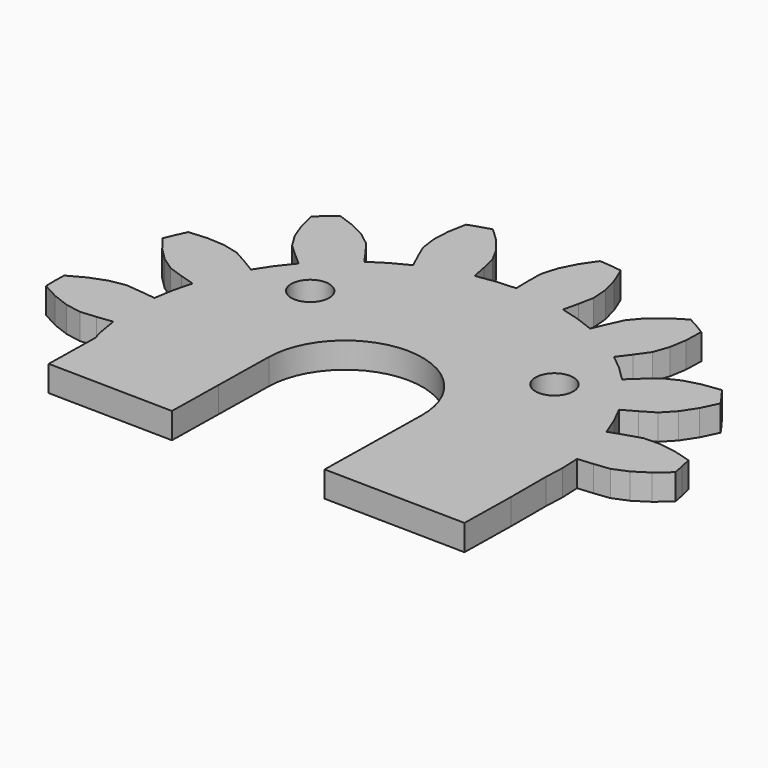
from build123d import *

# Parameters (mm, degrees)
F1_DEPTH  = 1.5
F2_R      = 1.1
F3_DEPTH  = 1.5
F4_W      = 4.2642379355
F4_H      = 1.5
F4_W_2    = 3
F4_W_3    = 5.2441455437
F3_FACE_W = 8.0745559603
F3_FACE_H = 1.5
F5_DEPTH  = 3.3


with BuildPart() as f1:
    # F0 (on Top) → F1 (new body)
    with BuildSketch(Plane.XY):
        Polygon((12.573339, -1.121183), (12.623723, 0), (12.573339, 1.121183), (13.469712, 1.201909), (14.363964, 1.305965), (15.232179, 1.665703), (16.071924, 2.205645), (16.876276, 2.889975), (16.752232, 3.534499), (16.603401, 4.173754), (15.590247, 4.47176), (14.603487, 4.623467), (13.664014, 4.59897), (12.804751, 4.330305), (11.95304, 4.039463), (11.543041, 5.084208), (11.040987, 6.087967), (11.82703, 6.526301), (12.601647, 6.985086), (13.248481, 7.666858), (13.796013, 8.501675), (14.252483, 9.454001), (13.877012, 9.992349), (13.481039, 10.515803), (12.434267, 10.375958), (11.471112, 10.113197), (10.622825, 9.7087), (9.947125, 9.113769), (9.287344, 8.50165), (8.487856, 9.28931), (7.620941, 10.002086), (8.16074, 10.722236), (8.681783, 11.456422), (8.995394, 12.342344), (9.156039, 13.327688), (9.185699, 14.383344), (8.623723, 14.722432), (8.049076, 15.039574), (7.149682, 14.486059), (6.376671, 13.854265), (5.766246, 13.139708), (5.390943, 12.321379), (5.037175, 11.493824), (3.986435, 11.888206), (2.904557, 12.186753), (3.104777, 13.0642), (3.282153, 13.946839), (3.208314, 14.883726), (2.954295, 15.849223), (2.552017, 16.825676), (1.900707, 16.906872), (1.246748, 16.962866), (0.650245, 16.091388), (0.201038, 15.199803), (-0.065977, 14.298742), (-0.075988, 13.398512), (-0.062575, 12.498612), (-1.182883, 12.431524), (-2.292658, 12.264221), (-2.466637, 13.147244), (-2.663598, 14.025721), (-3.112119, 14.851577), (-3.736881, 15.630283), (-4.501539, 16.358696), (-5.129566, 16.167961), (-5.749762, 15.953124), (-5.940233, 14.91437), (-5.987963, 13.917158), (-5.865399, 12.985393), (-5.508388, 12.15892), (-5.130112, 11.342276), (-6.126277, 10.825318), (-7.072058, 10.221092), (-7.590155, 10.957011), (-8.127396, 11.679428), (-8.873046, 12.251455), (-9.760523, 12.708725), (-10.755346, 13.063149), (-11.251497, 12.633462), (-11.730693, 12.184943), (-11.482197, 11.158522), (-11.120198, 10.22811), (-10.629247, 9.426751), (-9.966945, 8.81694), (-9.289213, 8.224757), (-9.988989, 7.347316), (-10.607243, 6.410645), (-11.379873, 6.872211), (-12.164501, 7.313656), (-13.07835, 7.532945), (-14.075089, 7.589713), (-15.128062, 7.508865), (-15.40655, 6.914523), (-15.661887, 6.309874), (-15.017392, 5.473264), (-14.308257, 4.770528), (-13.533809, 4.238139), (-12.680733, 3.950431), (-11.820732, 3.685104), (-12.103122, 2.598896), (-12.286947, 1.491738), (-13.180515, 1.599143), (-14.07686, 1.683286), (-15.000896, 1.511921), (-15.934551, 1.158371), (-16.863606, 0.656229), (-16.876277, 0), (-16.863606, -0.656229), (-15.934551, -1.158371), (-15.000896, -1.511921), (-14.07686, -1.683286), (-13.180515, -1.599143), (-12.286947, -1.491738), (-12.103122, -2.598896), (-11.820732, -3.685104), (-12.680733, -3.950431), (-13.533809, -4.238139), (-14.308257, -4.770528), (-15.017392, -5.473264), (-15.661887, -6.309874), (-15.40655, -6.914523), (-15.128062, -7.508865), (-14.075089, -7.589713), (-13.07835, -7.532945), (-12.164501, -7.313656), (-11.379873, -6.872211), (-10.607243, -6.410645), (-9.988989, -7.347316), (-9.289213, -8.224757), (-9.966945, -8.81694), (-10.629247, -9.426751), (-11.120198, -10.22811), (-11.482197, -11.158522), (-11.730693, -12.184943), (-11.251497, -12.633462), (-10.755346, -13.063149), (-9.760523, -12.708725), (-8.873046, -12.251455), (-8.127396, -11.679428), (-7.590155, -10.957011), (-7.072058, -10.221092), (-6.126277, -10.825318), (-5.130112, -11.342276), (-5.508388, -12.15892), (-5.865399, -12.985393), (-5.987963, -13.917158), (-5.940233, -14.91437), (-5.749762, -15.953124), (-5.129566, -16.167961), (-4.501539, -16.358696), (-3.736881, -15.630283), (-3.112119, -14.851577), (-2.663598, -14.025721), (-2.466637, -13.147244), (-2.292658, -12.264221), (-1.182883, -12.431524), (-0.062575, -12.498612), (-0.075988, -13.398512), (-0.065977, -14.298742), (0.201038, -15.199803), (0.650245, -16.091388), (1.246748, -16.962866), (1.900707, -16.906872), (2.552017, -16.825676), (2.954295, -15.849223), (3.208314, -14.883726), (3.282153, -13.946839), (3.104777, -13.0642), (2.904557, -12.186753), (3.986435, -11.888206), (5.037175, -11.493824), (5.390943, -12.321379), (5.766246, -13.139708), (6.376671, -13.854265), (7.149682, -14.486059), (8.049076, -15.039574), (8.623723, -14.722432), (9.185699, -14.383344), (9.156039, -13.327688), (8.995394, -12.342344), (8.681783, -11.456422), (8.16074, -10.722236), (7.620941, -10.002086), (8.487856, -9.28931), (9.287344, -8.50165), (9.947125, -9.113769), (10.622825, -9.7087), (11.471112, -10.113197), (12.434267, -10.375958), (13.481039, -10.515803), (13.877012, -9.992349), (14.252483, -9.454001), (13.796013, -8.501675), (13.248481, -7.666858), (12.601647, -6.985086), (11.82703, -6.526301), (11.040987, -6.087967), (11.543041, -5.084208), (11.95304, -4.039463), (12.804751, -4.330305), (13.664014, -4.59897), (14.603487, -4.623467), (15.590247, -4.47176), (16.603401, -4.173754), (16.752232, -3.534499), (16.876276, -2.889975), (16.071924, -2.205645), (15.232179, -1.665703), (14.363964, -1.305965), (13.469712, -1.201909), align=None)
    extrude(amount=F1_DEPTH)

    # F2 (on face) → F3 (cut, through all)
    with BuildSketch(Plane.XY.offset(1.5)):
        with Locations((-7.1978296976, 6.45)):
            Circle(F2_R)
        with Locations((7.2, 6.2)):
            Circle(F2_R)
        with BuildLine():
            Line((13.469712, -1.201909), (12.573339, -1.121183))
            Line((12.573339, -1.121183), (12.573339, -3.685104))
            Line((12.573339, -3.685104), (4.5, -3.5449207368))
            Line((4.5, -3.5449207368), (4.330384853, -3.5449207368))
            Line((4.330384853, -3.5449207368), (4.3927680428, 0.0478094358))
            ThreePointArc((4.3927680428, 0.0478094358), (-0.0284287377, 4.6252562163), (-4.6058755182, 0.2040594358))
            Line((-4.6058755182, 0.2040594358), (-4.6682075846, -3.3857264732))
            Line((-4.6682075846, -3.3857264732), (-11.9313506872, -3.2596112313))
            Line((-11.9313506872, -3.2596112313), (-11.820732, -3.685104))
            Line((-11.820732, -3.685104), (-12.680733, -3.950431))
            Line((-12.680733, -3.950431), (-13.533809, -4.238139))
            Line((-13.533809, -4.238139), (-14.308257, -4.770528))
            Line((-14.308257, -4.770528), (-15.017392, -5.473264))
            Line((-15.017392, -5.473264), (-15.661887, -6.309874))
            Line((-15.661887, -6.309874), (-15.40655, -6.914523))
            Line((-15.40655, -6.914523), (-15.128062, -7.508865))
            Line((-15.128062, -7.508865), (-14.075089, -7.589713))
            Line((-14.075089, -7.589713), (-13.07835, -7.532945))
            Line((-13.07835, -7.532945), (-12.164501, -7.313656))
            Line((-12.164501, -7.313656), (-11.379873, -6.872211))
            Line((-11.379873, -6.872211), (-10.607243, -6.410645))
            Line((-10.607243, -6.410645), (-9.988989, -7.347316))
            Line((-9.988989, -7.347316), (-9.289213, -8.224757))
            Line((-9.289213, -8.224757), (-9.966945, -8.81694))
            Line((-9.966945, -8.81694), (-10.629247, -9.426751))
            Line((-10.629247, -9.426751), (-11.120198, -10.22811))
            Line((-11.120198, -10.22811), (-11.482197, -11.158522))
            Line((-11.482197, -11.158522), (-11.730693, -12.184943))
            Line((-11.730693, -12.184943), (-11.251497, -12.633462))
            Line((-11.251497, -12.633462), (-10.755346, -13.063149))
            Line((-10.755346, -13.063149), (-9.760523, -12.708725))
            Line((-9.760523, -12.708725), (-8.873046, -12.251455))
            Line((-8.873046, -12.251455), (-8.127396, -11.679428))
            Line((-8.127396, -11.679428), (-7.590155, -10.957011))
            Line((-7.590155, -10.957011), (-7.072058, -10.221092))
            Line((-7.072058, -10.221092), (-6.126277, -10.825318))
            Line((-6.126277, -10.825318), (-5.130112, -11.342276))
            Line((-5.130112, -11.342276), (-5.508388, -12.15892))
            Line((-5.508388, -12.15892), (-5.865399, -12.985393))
            Line((-5.865399, -12.985393), (-5.987963, -13.917158))
            Line((-5.987963, -13.917158), (-5.940233, -14.91437))
            Line((-5.940233, -14.91437), (-5.749762, -15.953124))
            Line((-5.749762, -15.953124), (-5.129566, -16.167961))
            Line((-5.129566, -16.167961), (-4.501539, -16.358696))
            Line((-4.501539, -16.358696), (-3.736881, -15.630283))
            Line((-3.736881, -15.630283), (-3.112119, -14.851577))
            Line((-3.112119, -14.851577), (-2.663598, -14.025721))
            Line((-2.663598, -14.025721), (-2.466637, -13.147244))
            Line((-2.466637, -13.147244), (-2.292658, -12.264221))
            Line((-2.292658, -12.264221), (-1.182883, -12.431524))
            Line((-1.182883, -12.431524), (-0.062575, -12.498612))
            Line((-0.062575, -12.498612), (-0.075988, -13.398512))
            Line((-0.075988, -13.398512), (-0.065977, -14.298742))
            Line((-0.065977, -14.298742), (0.201038, -15.199803))
            Line((0.201038, -15.199803), (0.650245, -16.091388))
            Line((0.650245, -16.091388), (1.246748, -16.962866))
            Line((1.246748, -16.962866), (1.900707, -16.906872))
            Line((1.900707, -16.906872), (2.552017, -16.825676))
            Line((2.552017, -16.825676), (2.954295, -15.849223))
            Line((2.954295, -15.849223), (3.208314, -14.883726))
            Line((3.208314, -14.883726), (3.282153, -13.946839))
            Line((3.282153, -13.946839), (3.104777, -13.0642))
            Line((3.104777, -13.0642), (2.904557, -12.186753))
            Line((2.904557, -12.186753), (3.986435, -11.888206))
            Line((3.986435, -11.888206), (5.037175, -11.493824))
            Line((5.037175, -11.493824), (5.390943, -12.321379))
            Line((5.390943, -12.321379), (5.766246, -13.139708))
            Line((5.766246, -13.139708), (6.376671, -13.854265))
            Line((6.376671, -13.854265), (7.149682, -14.486059))
            Line((7.149682, -14.486059), (8.049076, -15.039574))
            Line((8.049076, -15.039574), (8.623723, -14.722432))
            Line((8.623723, -14.722432), (9.185699, -14.383344))
            Line((9.185699, -14.383344), (9.156039, -13.327688))
            Line((9.156039, -13.327688), (8.995394, -12.342344))
            Line((8.995394, -12.342344), (8.681783, -11.456422))
            Line((8.681783, -11.456422), (8.16074, -10.722236))
            Line((8.16074, -10.722236), (7.620941, -10.002086))
            Line((7.620941, -10.002086), (8.487856, -9.28931))
            Line((8.487856, -9.28931), (9.287344, -8.50165))
            Line((9.287344, -8.50165), (9.947125, -9.113769))
            Line((9.947125, -9.113769), (10.622825, -9.7087))
            Line((10.622825, -9.7087), (11.471112, -10.113197))
            Line((11.471112, -10.113197), (12.434267, -10.375958))
            Line((12.434267, -10.375958), (13.481039, -10.515803))
            Line((13.481039, -10.515803), (13.877012, -9.992349))
            Line((13.877012, -9.992349), (14.252483, -9.454001))
            Line((14.252483, -9.454001), (13.796013, -8.501675))
            Line((13.796013, -8.501675), (13.248481, -7.666858))
            Line((13.248481, -7.666858), (12.601647, -6.985086))
            Line((12.601647, -6.985086), (11.82703, -6.526301))
            Line((11.82703, -6.526301), (11.040987, -6.087967))
            Line((11.040987, -6.087967), (11.543041, -5.084208))
            Line((11.543041, -5.084208), (11.95304, -4.039463))
            Line((11.95304, -4.039463), (12.804751, -4.330305))
            Line((12.804751, -4.330305), (13.664014, -4.59897))
            Line((13.664014, -4.59897), (14.603487, -4.623467))
            Line((14.603487, -4.623467), (15.590247, -4.47176))
            Line((15.590247, -4.47176), (16.603401, -4.173754))
            Line((16.603401, -4.173754), (16.752232, -3.534499))
            Line((16.752232, -3.534499), (16.876276, -2.889975))
            Line((16.876276, -2.889975), (16.071924, -2.205645))
            Line((16.071924, -2.205645), (15.232179, -1.665703))
            Line((15.232179, -1.665703), (14.363964, -1.305965))
            Line((14.363964, -1.305965), (13.469712, -1.201909))
        make_face()
    extrude(amount=-F3_DEPTH, mode=Mode.SUBTRACT)

    # F4 (on face) + F3_face (on face) → F5 (join)
    with BuildSketch(Plane(origin=(-0.0601781504, -3.4657390433, 0), x_dir=(0.9998492846, -0.0173611111, 0), z_dir=(-0.0173611111, -0.9998492846, 0))):
        with Locations((-6.7408430078, 0.75)):
            Rectangle(F4_W, F4_H)
        with Locations((-10.3729619756, 0.75)):
            Rectangle(F4_W_2, F4_H)
        with Locations((7.0133487317, 0.75)):
            Rectangle(F4_W_3, F4_H)
    with BuildSketch(Plane(origin=(-8.2997791359, -3.3226688522, 0.75), x_dir=(0.9998492846, -0.0173611111, 0), z_dir=(-0.0173611111, -0.9998492846, 0))):
        with Locations((16.8389865313, 0)):
            Rectangle(F3_FACE_W, F3_FACE_H)
    extrude(amount=F5_DEPTH)


solid = f1.part
